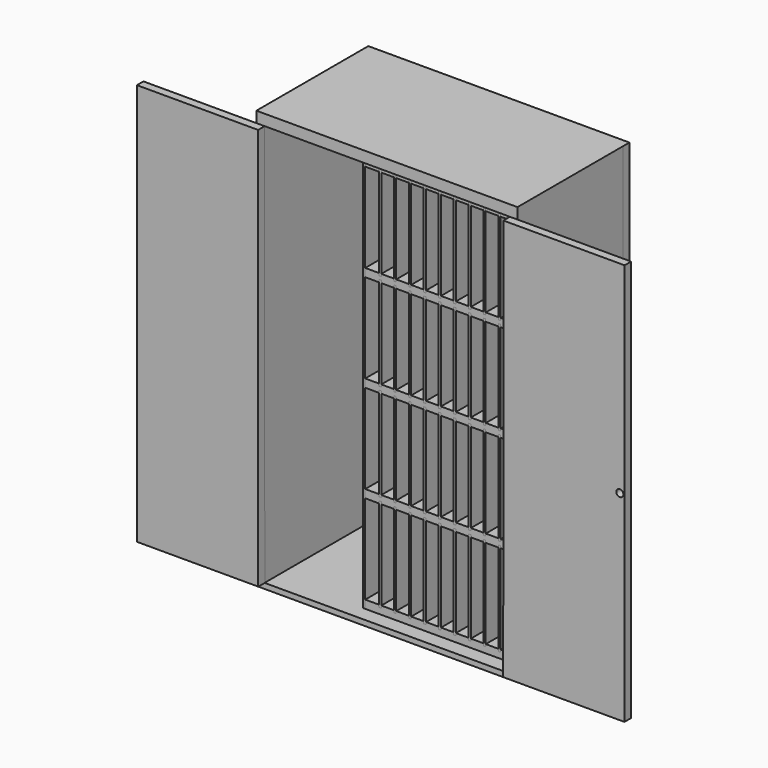
from build123d import *

# Parameters (mm, degrees)
F1_DEPTH      = 330.2
F2_W          = 6.35
F2_H          = 0.635
F3_DEPTH      = 254
F2_H_2        = 0.3175
F2_H_3        = 0.9525
F2_H_4        = 1081.5688967705
F4_W          = 711.1986837864
F4_H          = 1139.7287186623
F4_W_2        = 666.7486837864
F4_H_2        = 1095.2787186623
F5_DEPTH      = 355.6
F5_DEPTH_BACK = 25.4
F7_W          = 711.1986837864
F7_H          = 1139.7287186623
F7_R          = 25.4
F8_DEPTH      = 22.225
F9_DEPTH      = 25.4
F11_R         = 9.525
F12_DEPTH     = 22.225


# Not quite as in the source:
# - a feature names something its author has since deleted; it is built from what else it names


with BuildPart() as f1:
    # F0 (on Front) → F1 (new body)
    with BuildSketch(Plane.XZ):
        Polygon((43.8150024557, 510.2225423241), (43.8150024557, 503.8725423241), (78.1050024557, 503.8725423241), (78.1050024557, 510.2225423241), (84.4550024557, 510.2225423241), (84.4550024557, 503.8725423241), (118.7450024557, 503.8725423241), (118.7450024557, 510.2225423241), (125.0950024557, 510.2225423241), (125.0950024557, 503.8725423241), (159.3850024557, 503.8725423241), (159.3850024557, 510.2225423241), (165.7350024557, 510.2225423241), (165.7350024557, 503.8725423241), (203.2000024557, 503.8725423241), (203.2000024557, 526.0975423241), (-203.1999975443, 526.0975423241), (-203.1999975443, 503.8725423241), (-165.7349975443, 503.8725423241), (-165.7349975443, 510.2225423241), (-159.3849975443, 510.2225423241), (-159.3849975443, 503.8725423241), (-125.0949975443, 503.8725423241), (-125.0949975443, 510.2225423241), (-118.7449975443, 510.2225423241), (-118.7449975443, 503.8725423241), (-84.4549975443, 503.8725423241), (-84.4549975443, 510.2225423241), (-78.1049975443, 510.2225423241), (-78.1049975443, 503.8725423241), (-43.8149975443, 503.8725423241), (-43.8149975443, 510.2225423241), (-37.4649975443, 510.2225423241), (-37.4649975443, 503.8725423241), (-3.1749975443, 503.8725423241), (-3.1749975443, 510.2225423241), (3.1750024557, 510.2225423241), (3.1750024557, 503.8725423241), (37.4650024557, 503.8725423241), (37.4650024557, 510.2225423241), align=None)
    extrude(amount=-F1_DEPTH)

    # F7 (on offset) → F9 (cut)
    with BuildSketch(Plane(origin=(0, 355.6, 0), x_dir=(-1, 0, 0), z_dir=(0, 1, 0))):
        with Locations((431.7003317833, -533.4750243187)):
            Circle(F7_R)
    extrude(amount=-F9_DEPTH, mode=Mode.SUBTRACT)


with BuildPart() as f1b:
    # F0 (on Front) → F1, piece 2 (new body)
    with BuildSketch(Plane.XZ):
        Polygon((-203.1999975443, 260.9850423241), (-203.1999975443, 238.7600423241), (-165.7349975443, 238.7600423241), (-165.7349975443, 245.1100423241), (-159.3849975443, 245.1100423241), (-159.3849975443, 238.7600423241), (-125.0949975443, 238.7600423241), (-125.0949975443, 245.1100423241), (-118.7449975443, 245.1100423241), (-118.7449975443, 238.7600423241), (-84.4549975443, 238.7600423241), (-84.4549975443, 245.1100423241), (-78.1049975443, 245.1100423241), (-78.1049975443, 238.7600423241), (-43.8149975443, 238.7600423241), (-43.8149975443, 245.1100423241), (-37.4649975443, 245.1100423241), (-37.4649975443, 238.7600423241), (-3.1749975443, 238.7600423241), (-3.1749975443, 245.1100423241), (3.1750024557, 245.1100423241), (3.1750024557, 238.7600423241), (37.4650024557, 238.7600423241), (37.4650024557, 245.1100423241), (43.8150024557, 245.1100423241), (43.8150024557, 238.7600423241), (78.1050024557, 238.7600423241), (78.1050024557, 245.1100423241), (84.4550024557, 245.1100423241), (84.4550024557, 238.7600423241), (118.7450024557, 238.7600423241), (118.7450024557, 245.1100423241), (125.0950024557, 245.1100423241), (125.0950024557, 238.7600423241), (159.3850024557, 238.7600423241), (159.3850024557, 245.1100423241), (165.7350024557, 245.1100423241), (165.7350024557, 238.7600423241), (203.2000024557, 238.7600423241), (203.2000024558, 260.9850423241), (165.7350024557, 260.9850423241), (165.7350024557, 254.6350423241), (159.3850024557, 254.6350423241), (159.3850024557, 260.9850423241), (125.0950024557, 260.9850423241), (125.0950024557, 254.6350423241), (118.7450024557, 254.6350423241), (118.7450024557, 260.9850423241), (84.4550024557, 260.9850423241), (84.4550024557, 254.6350423241), (78.1050024557, 254.6350423241), (78.1050024557, 260.9850423241), (43.8150024557, 260.9850423241), (43.8150024557, 254.6350423241), (37.4650024557, 254.6350423241), (37.4650024557, 260.9850423241), (3.1750024557, 260.9850423241), (3.1750024557, 254.6350423241), (-3.1749975443, 254.6350423241), (-3.1749975443, 260.9850423241), (-37.4649975443, 260.9850423241), (-37.4649975443, 254.6350423241), (-43.8149975443, 254.6350423241), (-43.8149975443, 260.9850423241), (-78.1049975443, 260.9850423241), (-78.1049975443, 254.6350423241), (-84.4549975443, 254.6350423241), (-84.4549975443, 260.9850423241), (-118.7449975443, 260.9850423241), (-118.7449975443, 254.6350423241), (-125.0949975443, 254.6350423241), (-125.0949975443, 260.9850423241), (-159.3849975443, 260.9850423241), (-159.3849975443, 254.6350423241), (-165.7349975443, 254.6350423241), (-165.7349975443, 260.9850423241), align=None)
    extrude(amount=-F1_DEPTH)


with BuildPart() as f1c:
    # F0 (on Front) → F1, piece 3 (new body)
    with BuildSketch(Plane.XZ):
        Polygon((-203.1999975443, -4.1274576759), (-203.1999975443, -26.3524576759), (-165.7349975443, -26.3524576759), (-165.7349975443, -20.0024576759), (-159.3849975443, -20.0024576759), (-159.3849975443, -26.3524576759), (-125.0949975443, -26.3524576759), (-125.0949975443, -20.0024576759), (-118.7449975443, -20.0024576759), (-118.7449975443, -26.3524576759), (-84.4549975443, -26.3524576759), (-84.4549975443, -20.0024576759), (-78.1049975443, -20.0024576759), (-78.1049975443, -26.3524576759), (-43.8149975443, -26.3524576759), (-43.8149975443, -20.0024576759), (-37.4649975443, -20.0024576759), (-37.4649975443, -26.3524576759), (-3.1749975443, -26.3524576759), (-3.1749975443, -20.0024576759), (3.1750024557, -20.0024576759), (3.1750024557, -26.3524576759), (37.4650024557, -26.3524576759), (37.4650024557, -20.0024576759), (43.8150024557, -20.0024576759), (43.8150024557, -26.3524576759), (78.1050024557, -26.3524576759), (78.1050024557, -20.0024576759), (84.4550024557, -20.0024576759), (84.4550024557, -26.3524576759), (118.7450024557, -26.3524576759), (118.7450024557, -20.0024576759), (125.0950024557, -20.0024576759), (125.0950024557, -26.3524576759), (159.3850024557, -26.3524576759), (159.3850024557, -20.0024576759), (165.7350024557, -20.0024576759), (165.7350024557, -26.3524576759), (203.2000024557, -26.3524576759), (203.2000024558, -4.1274576759), (165.7350024557, -4.1274576759), (165.7350024557, -10.4774576759), (159.3850024557, -10.4774576759), (159.3850024557, -4.1274576759), (125.0950024557, -4.1274576759), (125.0950024557, -10.4774576759), (118.7450024557, -10.4774576759), (118.7450024557, -4.1274576759), (84.4550024557, -4.1274576759), (84.4550024557, -10.4774576759), (78.1050024557, -10.4774576759), (78.1050024557, -4.1274576759), (43.8150024557, -4.1274576759), (43.8150024557, -10.4774576759), (37.4650024557, -10.4774576759), (37.4650024557, -4.1274576759), (3.1750024557, -4.1274576759), (3.1750024557, -10.4774576759), (-3.1749975443, -10.4774576759), (-3.1749975443, -4.1274576759), (-37.4649975443, -4.1274576759), (-37.4649975443, -10.4774576759), (-43.8149975443, -10.4774576759), (-43.8149975443, -4.1274576759), (-78.1049975443, -4.1274576759), (-78.1049975443, -10.4774576759), (-84.4549975443, -10.4774576759), (-84.4549975443, -4.1274576759), (-118.7449975443, -4.1274576759), (-118.7449975443, -10.4774576759), (-125.0949975443, -10.4774576759), (-125.0949975443, -4.1274576759), (-159.3849975443, -4.1274576759), (-159.3849975443, -10.4774576759), (-165.7349975443, -10.4774576759), (-165.7349975443, -4.1274576759), align=None)
    extrude(amount=-F1_DEPTH)


with BuildPart() as f1d:
    # F0 (on Front) → F1, piece 4 (new body)
    with BuildSketch(Plane.XZ):
        Polygon((118.7450024557, -275.5899576759), (118.7450024557, -269.2399576759), (84.4550024557, -269.2399576759), (84.4550024557, -275.5899576759), (78.1050024557, -275.5899576759), (78.1050024557, -269.2399576759), (43.8150024557, -269.2399576759), (43.8150024557, -275.5899576759), (37.4650024557, -275.5899576759), (37.4650024557, -269.2399576759), (3.1750024557, -269.2399576759), (3.1750024557, -275.5899576759), (-3.1749975443, -275.5899576759), (-3.1749975443, -269.2399576759), (-37.4649975443, -269.2399576759), (-37.4649975443, -275.5899576759), (-43.8149975443, -275.5899576759), (-43.8149975443, -269.2399576759), (-78.1049975443, -269.2399576759), (-78.1049975443, -275.5899576759), (-84.4549975443, -275.5899576759), (-84.4549975443, -269.2399576759), (-118.7449975443, -269.2399576759), (-118.7449975443, -275.5899576759), (-125.0949975443, -275.5899576759), (-125.0949975443, -269.2399576759), (-159.3849975443, -269.2399576759), (-159.3849975443, -275.5899576759), (-165.7349975443, -275.5899576759), (-165.7349975443, -269.2399576759), (-203.1999975443, -269.2399576759), (-203.1999975443, -291.4649576759), (-165.7349975443, -291.4649576759), (-165.7349975443, -285.1149576759), (-159.3849975443, -285.1149576759), (-159.3849975443, -291.4649576759), (-125.0949975443, -291.4649576759), (-125.0949975443, -285.1149576759), (-118.7449975443, -285.1149576759), (-118.7449975443, -291.4649576759), (-84.4549975443, -291.4649576759), (-84.4549975443, -285.1149576759), (-78.1049975443, -285.1149576759), (-78.1049975443, -291.4649576759), (-43.8149975443, -291.4649576759), (-43.8149975443, -285.1149576759), (-37.4649975443, -285.1149576759), (-37.4649975443, -291.4649576759), (-3.1749975443, -291.4649576759), (-3.1749975443, -285.1149576759), (3.1750024557, -285.1149576759), (3.1750024557, -291.4649576759), (37.4650024557, -291.4649576759), (37.4650024557, -285.1149576759), (43.8150024557, -285.1149576759), (43.8150024557, -291.4649576759), (78.1050024557, -291.4649576759), (78.1050024557, -285.1149576759), (84.4550024557, -285.1149576759), (84.4550024557, -291.4649576759), (118.7450024557, -291.4649576759), (118.7450024557, -285.1149576759), (125.0950024557, -285.1149576759), (125.0950024557, -291.4649576759), (159.3850024557, -291.4649576759), (159.3850024557, -285.1149576759), (165.7350024557, -285.1149576759), (165.7350024557, -291.4649576759), (203.2000024557, -291.4649576759), (203.2000024558, -269.2399576759), (165.7350024557, -269.2399576759), (165.7350024557, -275.5899576759), (159.3850024557, -275.5899576759), (159.3850024557, -269.2399576759), (125.0950024557, -269.2399576759), (125.0950024557, -275.5899576759), align=None)
    extrude(amount=-F1_DEPTH)


with BuildPart() as f1e:
    # F0 (on Front) → F1, piece 5 (new body)
    with BuildSketch(Plane.XZ):
        Polygon((-203.1999975443, -556.5774576759), (203.2000024557, -556.5774576759), (203.2000024557, -534.3524576759), (165.7350024557, -534.3524576759), (165.7350024557, -540.7024576759), (159.3850024557, -540.7024576759), (159.3850024557, -534.3524576759), (125.0950024557, -534.3524576759), (125.0950024557, -540.7024576759), (118.7450024557, -540.7024576759), (118.7450024557, -534.3524576759), (84.4550024557, -534.3524576759), (84.4550024557, -540.7024576759), (78.1050024557, -540.7024576759), (78.1050024557, -534.3524576759), (43.8150024557, -534.3524576759), (43.8150024557, -540.7024576759), (37.4650024557, -540.7024576759), (37.4650024557, -534.3524576759), (3.1750024557, -534.3524576759), (3.1750024557, -540.7024576759), (-3.1749975443, -540.7024576759), (-3.1749975443, -534.3524576759), (-37.4649975443, -534.3524576759), (-37.4649975443, -540.7024576759), (-43.8149975443, -540.7024576759), (-43.8149975443, -534.3524576759), (-78.1049975443, -534.3524576759), (-78.1049975443, -540.7024576759), (-84.4549975443, -540.7024576759), (-84.4549975443, -534.3524576759), (-118.7449975443, -534.3524576759), (-118.7449975443, -540.7024576759), (-125.0949975443, -540.7024576759), (-125.0949975443, -534.3524576759), (-159.3849975443, -534.3524576759), (-159.3849975443, -540.7024576759), (-165.7349975443, -540.7024576759), (-165.7349975443, -534.3524576759), (-203.1999975443, -534.3524576759), align=None)
    extrude(amount=-F1_DEPTH)


with BuildPart() as f3:
    # F2 (on Front) → F3 (new body)
    with BuildSketch(Plane.XZ):
        with Locations((162.5600024557, -10.1599576759)):
            Rectangle(F2_W, F2_H)
        Polygon((159.3850024557, -4.1274576759), (159.3850024557, -9.8424576759), (165.7350024557, -9.8424576759), (165.7350024557, -4.1274576759), (165.7350024557, -3.4924576759), (165.7350024557, 238.7600423241), (165.7350024557, 239.3950423241), (165.7350024557, 245.1100423241), (159.3850024557, 245.1100423241), (159.3850024557, 239.3950423241), (159.3850024557, 238.7600423241), (159.3850024557, -3.4924576759), align=None)
        with Locations((162.5600024557, 245.4275423241)):
            Rectangle(F2_W, F2_H)
    extrude(amount=-F3_DEPTH)


with BuildPart() as f3b:
    # F2 (on Front) → F3, piece 2 (new body)
    with BuildSketch(Plane.XZ):
        Polygon((165.7350024557, -26.0349576759), (165.7350024557, -20.0024576759), (159.3850024557, -20.0024576759), (159.3850024557, -26.0349576759), (159.3850024557, -26.3524576759), (159.3850024557, -268.9224576759), (159.3850024557, -269.2399576759), (159.3850024557, -275.2724576759), (165.7350024557, -275.2724576759), (165.7350024557, -269.2399576759), (165.7350024557, -268.9224576759), (165.7350024557, -26.3524576759), align=None)
        with Locations((162.5600024557, -19.8437076759)):
            Rectangle(F2_W, F2_H_2)
        with Locations((162.5600024557, -275.4312076759)):
            Rectangle(F2_W, F2_H_2)
    extrude(amount=-F3_DEPTH)


with BuildPart() as f3c:
    # F2 (on Front) → F3, piece 3 (new body)
    with BuildSketch(Plane.XZ):
        with Locations((121.9200024557, -10.1599576759)):
            Rectangle(F2_W, F2_H)
        Polygon((118.7450024557, -4.1274576759), (118.7450024557, -9.8424576759), (125.0950024557, -9.8424576759), (125.0950024557, -4.1274576759), (125.0950024557, -3.4924576759), (125.0950024557, 238.7600423241), (125.0950024557, 239.3950423241), (125.0950024557, 245.1100423241), (118.7450024557, 245.1100423241), (118.7450024557, 239.3950423241), (118.7450024557, 238.7600423241), (118.7450024557, -3.4924576759), align=None)
        with Locations((121.9200024557, 245.4275423241)):
            Rectangle(F2_W, F2_H)
    extrude(amount=-F3_DEPTH)


with BuildPart() as f3d:
    # F2 (on Front) → F3, piece 4 (new body)
    with BuildSketch(Plane.XZ):
        Polygon((125.0950024557, -268.9224576759), (125.0950024557, -26.3524576759), (125.0950024557, -26.0349576759), (125.0950024557, -20.0024576759), (118.7450024557, -20.0024576759), (118.7450024557, -26.0349576759), (118.7450024557, -26.3524576759), (118.7450024557, -268.9224576759), (118.7450024557, -269.2399576759), (118.7450024557, -275.2724576759), (125.0950024557, -275.2724576759), (125.0950024557, -269.2399576759), align=None)
        with Locations((121.9200024557, -19.8437076759)):
            Rectangle(F2_W, F2_H_2)
        with Locations((121.9200024557, -275.4312076759)):
            Rectangle(F2_W, F2_H_2)
    extrude(amount=-F3_DEPTH)


with BuildPart() as f3e:
    # F2 (on Front) → F3, piece 5 (new body)
    with BuildSketch(Plane.XZ):
        with Locations((81.2800024557, -10.1599576759)):
            Rectangle(F2_W, F2_H)
        Polygon((78.1050024557, -4.1274576759), (78.1050024557, -9.8424576759), (84.4550024557, -9.8424576759), (84.4550024557, -4.1274576759), (84.4550024557, -3.4924576759), (84.4550024557, 238.7600423241), (84.4550024557, 239.3950423241), (84.4550024557, 245.1100423241), (78.1050024557, 245.1100423241), (78.1050024557, 239.3950423241), (78.1050024557, 238.7600423241), (78.1050024557, -3.4924576759), align=None)
        with Locations((81.2800024557, 245.4275423241)):
            Rectangle(F2_W, F2_H)
    extrude(amount=-F3_DEPTH)


with BuildPart() as f3f:
    # F2 (on Front) → F3, piece 6 (new body)
    with BuildSketch(Plane.XZ):
        Polygon((84.4550024557, -268.9224576759), (84.4550024557, -26.3524576759), (84.4550024557, -26.0349576759), (84.4550024557, -20.0024576759), (78.1050024557, -20.0024576759), (78.1050024557, -26.0349576759), (78.1050024557, -26.3524576759), (78.1050024557, -268.9224576759), (78.1050024557, -269.2399576759), (78.1050024557, -275.2724576759), (84.4550024557, -275.2724576759), (84.4550024557, -269.2399576759), align=None)
        with Locations((81.2800024557, -19.8437076759)):
            Rectangle(F2_W, F2_H_2)
        with Locations((81.2800024557, -275.4312076759)):
            Rectangle(F2_W, F2_H_2)
    extrude(amount=-F3_DEPTH)


with BuildPart() as f3g:
    # F2 (on Front) → F3, piece 7 (new body)
    with BuildSketch(Plane.XZ):
        with Locations((40.6400024557, -10.1599576759)):
            Rectangle(F2_W, F2_H)
        Polygon((37.4650024557, -4.1274576759), (37.4650024557, -9.8424576759), (43.8150024557, -9.8424576759), (43.8150024557, -4.1274576759), (43.8150024557, -3.4924576759), (43.8150024557, 238.7600423241), (43.8150024557, 239.3950423241), (43.8150024557, 245.1100423241), (37.4650024557, 245.1100423241), (37.4650024557, 239.3950423241), (37.4650024557, 238.7600423241), (37.4650024557, -3.4924576759), align=None)
        with Locations((40.6400024557, 245.4275423241)):
            Rectangle(F2_W, F2_H)
    extrude(amount=-F3_DEPTH)


with BuildPart() as f3h:
    # F2 (on Front) → F3, piece 8 (new body)
    with BuildSketch(Plane.XZ):
        Polygon((43.8150024557, -268.9224576759), (43.8150024557, -26.3524576759), (43.8150024557, -26.0349576759), (43.8150024557, -20.0024576759), (37.4650024557, -20.0024576759), (37.4650024557, -26.0349576759), (37.4650024557, -26.3524576759), (37.4650024557, -268.9224576759), (37.4650024557, -269.2399576759), (37.4650024557, -275.2724576759), (43.8150024557, -275.2724576759), (43.8150024557, -269.2399576759), align=None)
        with Locations((40.6400024557, -19.8437076759)):
            Rectangle(F2_W, F2_H_2)
        with Locations((40.6400024557, -275.4312076759)):
            Rectangle(F2_W, F2_H_2)
    extrude(amount=-F3_DEPTH)


with BuildPart() as f3i:
    # F2 (on Front) → F3, piece 9 (new body)
    with BuildSketch(Plane.XZ):
        with Locations((2.4557e-06, -10.1599576759)):
            Rectangle(F2_W, F2_H)
        Polygon((-3.1749975443, -4.1274576759), (-3.1749975443, -9.8424576759), (3.1750024557, -9.8424576759), (3.1750024557, -4.1274576759), (3.1750024557, -3.4924576759), (3.1750024557, 238.7600423241), (3.1750024557, 239.3950423241), (3.1750024557, 245.1100423241), (-3.1749975443, 245.1100423241), (-3.1749975443, 239.3950423241), (-3.1749975443, 238.7600423241), (-3.1749975443, -3.4924576759), align=None)
        with Locations((2.4557e-06, 245.4275423241)):
            Rectangle(F2_W, F2_H)
    extrude(amount=-F3_DEPTH)


with BuildPart() as f3j:
    # F2 (on Front) → F3, piece 10 (new body)
    with BuildSketch(Plane.XZ):
        Polygon((3.1750024557, -268.9224576759), (3.1750024557, -26.3524576759), (3.1750024557, -26.0349576759), (3.1750024557, -20.0024576759), (-3.1749975443, -20.0024576759), (-3.1749975443, -26.0349576759), (-3.1749975443, -26.3524576759), (-3.1749975443, -268.9224576759), (-3.1749975443, -269.2399576759), (-3.1749975443, -275.2724576759), (3.1750024557, -275.2724576759), (3.1750024557, -269.2399576759), align=None)
        with Locations((2.4557e-06, -19.8437076759)):
            Rectangle(F2_W, F2_H_2)
        with Locations((2.4557e-06, -275.4312076759)):
            Rectangle(F2_W, F2_H_2)
    extrude(amount=-F3_DEPTH)


with BuildPart() as f3k:
    # F2 (on Front) → F3, piece 11 (new body)
    with BuildSketch(Plane.XZ):
        with Locations((-40.6399975443, -10.1599576759)):
            Rectangle(F2_W, F2_H)
        Polygon((-43.8149975443, -4.1274576759), (-43.8149975443, -9.8424576759), (-37.4649975443, -9.8424576759), (-37.4649975443, -4.1274576759), (-37.4649975443, -3.4924576759), (-37.4649975443, 238.7600423241), (-37.4649975443, 239.3950423241), (-37.4649975443, 245.1100423241), (-43.8149975443, 245.1100423241), (-43.8149975443, 239.3950423241), (-43.8149975443, 238.7600423241), (-43.8149975443, -3.4924576759), align=None)
        with Locations((-40.6399975443, 245.4275423241)):
            Rectangle(F2_W, F2_H)
    extrude(amount=-F3_DEPTH)


with BuildPart() as f3l:
    # F2 (on Front) → F3, piece 12 (new body)
    with BuildSketch(Plane.XZ):
        Polygon((-37.4649975443, -268.9224576759), (-37.4649975443, -26.3524576759), (-37.4649975443, -26.0349576759), (-37.4649975443, -20.0024576759), (-43.8149975443, -20.0024576759), (-43.8149975443, -26.0349576759), (-43.8149975443, -26.3524576759), (-43.8149975443, -268.9224576759), (-43.8149975443, -269.2399576759), (-43.8149975443, -275.2724576759), (-37.4649975443, -275.2724576759), (-37.4649975443, -269.2399576759), align=None)
        with Locations((-40.6399975443, -19.8437076759)):
            Rectangle(F2_W, F2_H_2)
        with Locations((-40.6399975443, -275.4312076759)):
            Rectangle(F2_W, F2_H_2)
    extrude(amount=-F3_DEPTH)


with BuildPart() as f3m:
    # F2 (on Front) → F3, piece 13 (new body)
    with BuildSketch(Plane.XZ):
        with Locations((-81.2799975443, -10.1599576759)):
            Rectangle(F2_W, F2_H)
        Polygon((-84.4549975443, -4.1274576759), (-84.4549975443, -9.8424576759), (-78.1049975443, -9.8424576759), (-78.1049975443, -4.1274576759), (-78.1049975443, -3.4924576759), (-78.1049975443, 238.7600423241), (-78.1049975443, 239.3950423241), (-78.1049975443, 245.1100423241), (-84.4549975443, 245.1100423241), (-84.4549975443, 239.3950423241), (-84.4549975443, 238.7600423241), (-84.4549975443, -3.4924576759), align=None)
        with Locations((-81.2799975443, 245.4275423241)):
            Rectangle(F2_W, F2_H)
    extrude(amount=-F3_DEPTH)


with BuildPart() as f3n:
    # F2 (on Front) → F3, piece 14 (new body)
    with BuildSketch(Plane.XZ):
        Polygon((-78.1049975443, -268.9224576759), (-78.1049975443, -26.3524576759), (-78.1049975443, -26.0349576759), (-78.1049975443, -20.0024576759), (-84.4549975443, -20.0024576759), (-84.4549975443, -26.0349576759), (-84.4549975443, -26.3524576759), (-84.4549975443, -268.9224576759), (-84.4549975443, -269.2399576759), (-84.4549975443, -275.2724576759), (-78.1049975443, -275.2724576759), (-78.1049975443, -269.2399576759), align=None)
        with Locations((-81.2799975443, -19.8437076759)):
            Rectangle(F2_W, F2_H_2)
        with Locations((-81.2799975443, -275.4312076759)):
            Rectangle(F2_W, F2_H_2)
    extrude(amount=-F3_DEPTH)


with BuildPart() as f3o:
    # F2 (on Front) → F3, piece 15 (new body)
    with BuildSketch(Plane.XZ):
        with Locations((-121.9199975443, -10.1599576759)):
            Rectangle(F2_W, F2_H)
        Polygon((-125.0949975443, -4.1274576759), (-125.0949975443, -9.8424576759), (-118.7449975443, -9.8424576759), (-118.7449975443, -4.1274576759), (-118.7449975443, -3.4924576759), (-118.7449975443, 238.7600423241), (-118.7449975443, 239.3950423241), (-118.7449975443, 245.1100423241), (-125.0949975443, 245.1100423241), (-125.0949975443, 239.3950423241), (-125.0949975443, 238.7600423241), (-125.0949975443, -3.4924576759), align=None)
        with Locations((-121.9199975443, 245.4275423241)):
            Rectangle(F2_W, F2_H)
    extrude(amount=-F3_DEPTH)


with BuildPart() as f3p:
    # F2 (on Front) → F3, piece 16 (new body)
    with BuildSketch(Plane.XZ):
        Polygon((-118.7449975443, -268.9224576759), (-118.7449975443, -26.3524576759), (-118.7449975443, -26.0349576759), (-118.7449975443, -20.0024576759), (-125.0949975443, -20.0024576759), (-125.0949975443, -26.0349576759), (-125.0949975443, -26.3524576759), (-125.0949975443, -268.9224576759), (-125.0949975443, -269.2399576759), (-125.0949975443, -275.2724576759), (-118.7449975443, -275.2724576759), (-118.7449975443, -269.2399576759), align=None)
        with Locations((-121.9199975443, -19.8437076759)):
            Rectangle(F2_W, F2_H_2)
        with Locations((-121.9199975443, -275.4312076759)):
            Rectangle(F2_W, F2_H_2)
    extrude(amount=-F3_DEPTH)


with BuildPart() as f3q:
    # F2 (on Front) → F3, piece 17 (new body)
    with BuildSketch(Plane.XZ):
        with Locations((-162.5599975443, -10.1599576759)):
            Rectangle(F2_W, F2_H)
        Polygon((-165.7349975443, -4.1274576759), (-165.7349975443, -9.8424576759), (-159.3849975443, -9.8424576759), (-159.3849975443, -4.1274576759), (-159.3849975443, -3.4924576759), (-159.3849975443, 238.7600423241), (-159.3849975443, 239.3950423241), (-159.3849975443, 245.1100423241), (-165.7349975443, 245.1100423241), (-165.7349975443, 239.3950423241), (-165.7349975443, 238.7600423241), (-165.7349975443, -3.4924576759), align=None)
        with Locations((-162.5599975443, 245.4275423241)):
            Rectangle(F2_W, F2_H)
    extrude(amount=-F3_DEPTH)


with BuildPart() as f3r:
    # F2 (on Front) → F3, piece 18 (new body)
    with BuildSketch(Plane.XZ):
        Polygon((-159.3849975443, -268.9224576759), (-159.3849975443, -26.3524576759), (-159.3849975443, -26.0349576759), (-159.3849975443, -20.0024576759), (-165.7349975443, -20.0024576759), (-165.7349975443, -26.0349576759), (-165.7349975443, -26.3524576759), (-165.7349975443, -268.9224576759), (-165.7349975443, -269.2399576759), (-165.7349975443, -275.2724576759), (-159.3849975443, -275.2724576759), (-159.3849975443, -269.2399576759), align=None)
        with Locations((-162.5599975443, -19.8437076759)):
            Rectangle(F2_W, F2_H_2)
        with Locations((-162.5599975443, -275.4312076759)):
            Rectangle(F2_W, F2_H_2)
    extrude(amount=-F3_DEPTH)


with BuildPart() as f3s:
    # F2 (on Front) → F3, piece 19 (new body)
    with BuildSketch(Plane.XZ):
        Polygon((78.1050024557, -534.3524576759), (78.1050024557, -540.7024576759), (84.4550024557, -540.7024576759), (84.4550024557, -534.3524576759), (84.4550024557, -291.4649576759), (84.4550024557, -285.1149576759), (78.1050024557, -285.1149576759), (78.1050024557, -291.4649576759), align=None)
    extrude(amount=-F3_DEPTH)


with BuildPart() as f3t:
    # F2 (on Front) → F3, piece 20 (new body)
    with BuildSketch(Plane.XZ):
        Polygon((118.7450024557, -291.4649576759), (118.7450024557, -534.3524576759), (118.7450024557, -540.7024576759), (125.0950024557, -540.7024576759), (125.0950024557, -534.3524576759), (125.0950024557, -291.4649576759), (125.0950024557, -285.1149576759), (118.7450024557, -285.1149576759), align=None)
    extrude(amount=-F3_DEPTH)


with BuildPart() as f3u:
    # F2 (on Front) → F3, piece 21 (new body)
    with BuildSketch(Plane.XZ):
        Polygon((-165.7349975443, -534.3524576759), (-165.7349975443, -540.7024576759), (-159.3849975443, -540.7024576759), (-159.3849975443, -534.3524576759), (-159.3849975443, -291.4649576759), (-159.3849975443, -285.1149576759), (-165.7349975443, -285.1149576759), (-165.7349975443, -291.4649576759), align=None)
    extrude(amount=-F3_DEPTH)


with BuildPart() as f3v:
    # F2 (on Front) → F3, piece 22 (new body)
    with BuildSketch(Plane.XZ):
        Polygon((-84.4549975443, -540.7024576759), (-78.1049975443, -540.7024576759), (-78.1049975443, -534.3524576759), (-78.1049975443, -291.4649576759), (-78.1049975443, -285.1149576759), (-84.4549975443, -285.1149576759), (-84.4549975443, -291.4649576759), (-84.4549975443, -534.3524576759), align=None)
    extrude(amount=-F3_DEPTH)


with BuildPart() as f3w:
    # F2 (on Front) → F3, piece 23 (new body)
    with BuildSketch(Plane.XZ):
        Polygon((159.3850024557, -534.3524576759), (159.3850024557, -540.7024576759), (165.7350024557, -540.7024576759), (165.7350024557, -534.3524576759), (165.7350024557, -291.4649576759), (165.7350024557, -285.1149576759), (159.3850024557, -285.1149576759), (159.3850024557, -291.4649576759), align=None)
    extrude(amount=-F3_DEPTH)


with BuildPart() as f3x:
    # F2 (on Front) → F3, piece 24 (new body)
    with BuildSketch(Plane.XZ):
        Polygon((-3.1749975443, -540.7024576759), (3.1750024557, -540.7024576759), (3.1750024557, -534.3524576759), (3.1750024557, -291.4649576759), (3.1750024557, -285.1149576759), (-3.1749975443, -285.1149576759), (-3.1749975443, -291.4649576759), (-3.1749975443, -534.3524576759), align=None)
    extrude(amount=-F3_DEPTH)


with BuildPart() as f3y:
    # F2 (on Front) → F3, piece 25 (new body)
    with BuildSketch(Plane.XZ):
        Polygon((-125.0949975443, -534.3524576759), (-125.0949975443, -540.7024576759), (-118.7449975443, -540.7024576759), (-118.7449975443, -534.3524576759), (-118.7449975443, -291.4649576759), (-118.7449975443, -285.1149576759), (-125.0949975443, -285.1149576759), (-125.0949975443, -291.4649576759), align=None)
    extrude(amount=-F3_DEPTH)


with BuildPart() as f3z:
    # F2 (on Front) → F3, piece 26 (new body)
    with BuildSketch(Plane.XZ):
        Polygon((37.4650024557, -291.4649576759), (37.4650024557, -534.3524576759), (37.4650024557, -540.7024576759), (43.8150024557, -540.7024576759), (43.8150024557, -534.3524576759), (43.8150024557, -291.4649576759), (43.8150024557, -285.1149576759), (37.4650024557, -285.1149576759), align=None)
    extrude(amount=-F3_DEPTH)


with BuildPart() as f3ba:
    # F2 (on Front) → F3, piece 27 (new body)
    with BuildSketch(Plane.XZ):
        Polygon((-43.8149975443, -540.7024576759), (-37.4649975443, -540.7024576759), (-37.4649975443, -534.3524576759), (-37.4649975443, -291.4649576759), (-37.4649975443, -285.1149576759), (-43.8149975443, -285.1149576759), (-43.8149975443, -291.4649576759), (-43.8149975443, -534.3524576759), align=None)
    extrude(amount=-F3_DEPTH)


with BuildPart() as f3bb:
    # F2 (on Front) → F3, piece 28 (new body)
    with BuildSketch(Plane.XZ):
        Polygon((43.8150024557, 261.9375423241), (43.8150024557, 503.8725423241), (43.8150024557, 504.8250423241), (43.8150024557, 510.2225423241), (37.4650024557, 510.2225423241), (37.4650024557, 504.8250423241), (37.4650024557, 503.8725423241), (37.4650024557, 261.9375423241), (37.4650024557, 260.9850423241), (37.4650024557, 255.5875423241), (43.8150024557, 255.5875423241), (43.8150024557, 260.9850423241), align=None)
        with Locations((40.6400024557, 510.6987923241)):
            Rectangle(F2_W, F2_H_3)
        with Locations((40.6400024557, 255.1112923241)):
            Rectangle(F2_W, F2_H_3)
    extrude(amount=-F3_DEPTH)


with BuildPart() as f3bc:
    # F2 (on Front) → F3, piece 29 (new body)
    with BuildSketch(Plane.XZ):
        Polygon((-118.7449975443, 510.2225423241), (-125.0949975443, 510.2225423241), (-125.0949975443, 504.8250423241), (-125.0949975443, 503.8725423241), (-125.0949975443, 261.9375423241), (-125.0949975443, 260.9850423241), (-125.0949975443, 255.5875423241), (-118.7449975443, 255.5875423241), (-118.7449975443, 260.9850423241), (-118.7449975443, 261.9375423241), (-118.7449975443, 503.8725423241), (-118.7449975443, 504.8250423241), align=None)
        with Locations((-121.9199975443, 510.6987923241)):
            Rectangle(F2_W, F2_H_3)
        with Locations((-121.9199975443, 255.1112923241)):
            Rectangle(F2_W, F2_H_3)
    extrude(amount=-F3_DEPTH)


with BuildPart() as f3bd:
    # F2 (on Front) → F3, piece 30 (new body)
    with BuildSketch(Plane.XZ):
        Polygon((-37.4649975443, 261.9375423241), (-37.4649975443, 503.8725423241), (-37.4649975443, 504.8250423241), (-37.4649975443, 510.2225423241), (-43.8149975443, 510.2225423241), (-43.8149975443, 504.8250423241), (-43.8149975443, 503.8725423241), (-43.8149975443, 261.9375423241), (-43.8149975443, 260.9850423241), (-43.8149975443, 255.5875423241), (-37.4649975443, 255.5875423241), (-37.4649975443, 260.9850423241), align=None)
        with Locations((-40.6399975443, 510.6987923241)):
            Rectangle(F2_W, F2_H_3)
        with Locations((-40.6399975443, 255.1112923241)):
            Rectangle(F2_W, F2_H_3)
    extrude(amount=-F3_DEPTH)


with BuildPart() as f3be:
    # F2 (on Front) → F3, piece 31 (new body)
    with BuildSketch(Plane.XZ):
        Polygon((125.0950024557, 510.2225423241), (118.7450024557, 510.2225423241), (118.7450024557, 504.8250423241), (118.7450024557, 503.8725423241), (118.7450024557, 261.9375423241), (118.7450024557, 260.9850423241), (118.7450024557, 255.5875423241), (125.0950024557, 255.5875423241), (125.0950024557, 260.9850423241), (125.0950024557, 261.9375423241), (125.0950024557, 503.8725423241), (125.0950024557, 504.8250423241), align=None)
        with Locations((121.9200024557, 510.6987923241)):
            Rectangle(F2_W, F2_H_3)
        with Locations((121.9200024557, 255.1112923241)):
            Rectangle(F2_W, F2_H_3)
    extrude(amount=-F3_DEPTH)


with BuildPart() as f3bf:
    # F2 (on Front) → F3, piece 32 (new body)
    with BuildSketch(Plane.XZ):
        Polygon((84.4550024557, 510.2225423241), (78.1050024557, 510.2225423241), (78.1050024557, 504.8250423241), (78.1050024557, 503.8725423241), (78.1050024557, 261.9375423241), (78.1050024557, 260.9850423241), (78.1050024557, 255.5875423241), (84.4550024557, 255.5875423241), (84.4550024557, 260.9850423241), (84.4550024557, 261.9375423241), (84.4550024557, 503.8725423241), (84.4550024557, 504.8250423241), align=None)
        with Locations((81.2800024557, 510.6987923241)):
            Rectangle(F2_W, F2_H_3)
        with Locations((81.2800024557, 255.1112923241)):
            Rectangle(F2_W, F2_H_3)
    extrude(amount=-F3_DEPTH)


with BuildPart() as f3bg:
    # F2 (on Front) → F3, piece 33 (new body)
    with BuildSketch(Plane.XZ):
        Polygon((165.7350024557, 261.9375423241), (165.7350024557, 503.8725423241), (165.7350024557, 504.8250423241), (165.7350024557, 510.2225423241), (159.3850024557, 510.2225423241), (159.3850024557, 504.8250423241), (159.3850024557, 503.8725423241), (159.3850024557, 261.9375423241), (159.3850024557, 260.9850423241), (159.3850024557, 255.5875423241), (165.7350024557, 255.5875423241), (165.7350024557, 260.9850423241), align=None)
        with Locations((162.5600024557, 510.6987923241)):
            Rectangle(F2_W, F2_H_3)
        with Locations((162.5600024557, 255.1112923241)):
            Rectangle(F2_W, F2_H_3)
    extrude(amount=-F3_DEPTH)


with BuildPart() as f3bh:
    # F2 (on Front) → F3, piece 34 (new body)
    with BuildSketch(Plane.XZ):
        Polygon((-159.3849975443, 261.9375423241), (-159.3849975443, 503.8725423241), (-159.3849975443, 504.8250423241), (-159.3849975443, 510.2225423241), (-165.7349975443, 510.2225423241), (-165.7349975443, 504.8250423241), (-165.7349975443, 503.8725423241), (-165.7349975443, 261.9375423241), (-165.7349975443, 260.9850423241), (-165.7349975443, 255.5875423241), (-159.3849975443, 255.5875423241), (-159.3849975443, 260.9850423241), align=None)
        with Locations((-162.5599975443, 510.6987923241)):
            Rectangle(F2_W, F2_H_3)
        with Locations((-162.5599975443, 255.1112923241)):
            Rectangle(F2_W, F2_H_3)
    extrude(amount=-F3_DEPTH)


with BuildPart() as f3bi:
    # F2 (on Front) → F3, piece 35 (new body)
    with BuildSketch(Plane.XZ):
        Polygon((-78.1049975443, 261.9375423241), (-78.1049975443, 503.8725423241), (-78.1049975443, 504.8250423241), (-78.1049975443, 510.2225423241), (-84.4549975443, 510.2225423241), (-84.4549975443, 504.8250423241), (-84.4549975443, 503.8725423241), (-84.4549975443, 261.9375423241), (-84.4549975443, 260.9850423241), (-84.4549975443, 255.5875423241), (-78.1049975443, 255.5875423241), (-78.1049975443, 260.9850423241), align=None)
        with Locations((-81.2799975443, 510.6987923241)):
            Rectangle(F2_W, F2_H_3)
        with Locations((-81.2799975443, 255.1112923241)):
            Rectangle(F2_W, F2_H_3)
    extrude(amount=-F3_DEPTH)


with BuildPart() as f3bj:
    # F2 (on Front) → F3, piece 36 (new body)
    with BuildSketch(Plane.XZ):
        Polygon((3.1750024557, 504.8250423241), (3.1750024557, 510.2225423241), (-3.1749975443, 510.2225423241), (-3.1749975443, 504.8250423241), (-3.1749975443, 503.8725423241), (-3.1749975443, 261.9375423241), (-3.1749975443, 260.9850423241), (-3.1749975443, 255.5875423241), (3.1750024557, 255.5875423241), (3.1750024557, 260.9850423241), (3.1750024557, 261.9375423241), (3.1750024557, 503.8725423241), align=None)
        with Locations((2.4557e-06, 510.6987923241)):
            Rectangle(F2_W, F2_H_3)
        with Locations((2.4557e-06, 255.1112923241)):
            Rectangle(F2_W, F2_H_3)
    extrude(amount=-F3_DEPTH)


with BuildPart() as f3bk:
    # F2 (on Front) → F3, piece 37 (new body)
    with BuildSketch(Plane.XZ):
        with Locations((-206.3643879175, -15.8288776875)):
            Rectangle(F2_W, F2_H_4)
    extrude(amount=-F3_DEPTH)


with BuildPart() as f5:
    # F4 (on Front) → F5 (new body, two sides)
    with BuildSketch(Plane.XZ) as f5_sk:
        with Locations((-123.7428946018, -11.219650507)):
            Rectangle(F4_W, F4_H)
        with Locations((-123.7428946018, -18.7989179134)):
            Rectangle(F4_W_2, F4_H_2, mode=Mode.SUBTRACT)
    extrude(amount=-F5_DEPTH)
    extrude(f5_sk.sketch, amount=F5_DEPTH_BACK)

    # F7 (on offset) → F8 (join)
    with BuildSketch(Plane(origin=(0, 355.6, 0), x_dir=(-1, 0, 0), z_dir=(0, 1, 0))):
        with Locations((123.7302739382, -11.241105032)):
            Rectangle(F7_W, F7_H)
        with Locations((431.7003317833, -533.4750243187)):
            Circle(F7_R, mode=Mode.SUBTRACT)
    extrude(amount=-F8_DEPTH)

    # F11 (on offset) → F12 (join)
    with BuildSketch(Plane.XZ.offset(25.4)):
        Polygon((-456.5249979496, -566.302716732), (-456.8764567375, 528.7907719612), (-787.0764567375, 528.7907719612), (-786.7249979496, -566.302716732), align=None)
        Polygon((541.3635804176, 528.7907719612), (211.1635804176, 528.7907719612), (210.8121216297, -566.302716732), (541.0121216297, -566.302716732), align=None)
        with Locations((528.51190361, -21.7313145863)):
            Circle(F11_R, mode=Mode.SUBTRACT)
    extrude(amount=F12_DEPTH)


solid = Compound([f1.part, f1b.part, f1c.part, f1d.part, f1e.part, f3.part, f3b.part, f3c.part, f3d.part, f3e.part, f3f.part, f3g.part, f3h.part, f3i.part, f3j.part, f3k.part, f3l.part, f3m.part, f3n.part, f3o.part, f3p.part, f3q.part, f3r.part, f3s.part, f3t.part, f3u.part, f3v.part, f3w.part, f3x.part, f3y.part, f3z.part, f3ba.part, f3bb.part, f3bc.part, f3bd.part, f3be.part, f3bf.part, f3bg.part, f3bh.part, f3bi.part, f3bj.part, f3bk.part, f5.part])
